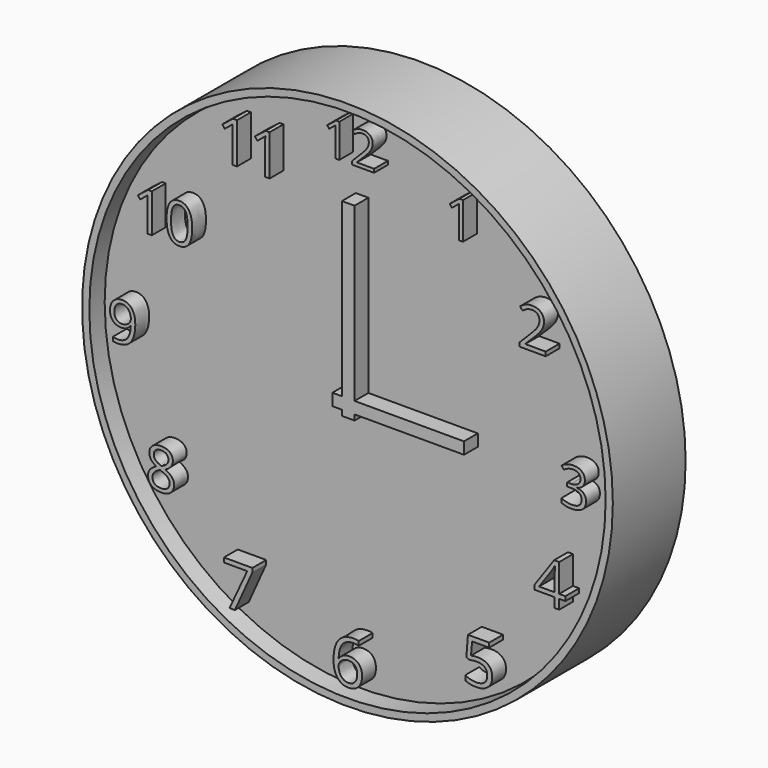
from build123d import *

# Parameters (mm, degrees)
F0_R            = 74.0699095202
F0_R_2          = 72.0569454693
F1_DEPTH        = 25.4
F2_R            = 71.6288838852
F3_DEPTH        = 20.574
F4_TEXT_SIZE    = 13.134137003
F4_TEXT_SIZE_2  = 14.3281546318
F4_TEXT_SIZE_3  = 15.5221670866
F4_TEXT_SIZE_4  = 14.7261585678
F4_TEXT_SIZE_5  = 16.3181736651
F4_TEXT_SIZE_6  = 16.7161795414
F4_TEXT_SIZE_7  = 16.7161847154
F4_TEXT_SIZE_8  = 15.5221722606
F4_TEXT_SIZE_9  = 15.1241631506
F4_TEXT_SIZE_10 = 15.1241612103
F4_TEXT_SIZE_11 = 15.9201729629
F4_TEXT_SIZE_12 = 17.1141854177
F5_DEPTH        = 25.4
F6_W            = 3.5199410049
F6_H            = 1.5269855503
F6_W_2          = 2.6841056533
F6_H_2          = 3.2999463147
F6_W_3          = 30.535359052
F6_H_3          = 47.972215456
F7_DEPTH        = 25.4


# Not quite as in the source:
# - Text() gives the source's letters only with a copy of the font that has no kerning and outlines rounded to 1/6400 em; it was checked with that copy


with BuildPart() as f1:
    # F0 (on Front) → F1 (new body)
    with BuildSketch(Plane.XZ):
        Circle(F0_R)
        Circle(F0_R_2, mode=Mode.SUBTRACT)
    extrude(amount=F1_DEPTH)


with BuildPart() as f3:
    # F2 (on Front) → F3 (new body)
    with BuildSketch(Plane.XZ):
        Circle(F2_R)
    extrude(amount=F3_DEPTH)

    # F4 (on Front) → F5 (join)
    with BuildSketch(Plane.XZ):
        with Locations((-6.8775145337, 59.4618432224)):
            Text('12', F4_TEXT_SIZE, font='Open Sans', text_align=(TextAlign.LEFT, TextAlign.BOTTOM))
        with Locations((27.2234939039, 50.5783893168)):
            Text('1', F4_TEXT_SIZE_2, font='Open Sans', text_align=(TextAlign.LEFT, TextAlign.BOTTOM))
        with Locations((47.2829155624, 29.9458447844)):
            Text('2', F4_TEXT_SIZE_3, font='Open Sans', text_align=(TextAlign.LEFT, TextAlign.BOTTOM))
        with Locations((59.0320006013, -5.0148512237)):
            Text('3', F4_TEXT_SIZE_4, font='Open Sans', text_align=(TextAlign.LEFT, TextAlign.BOTTOM))
        with Locations((51.8073847343, -31.0920923948)):
            Text('4', F4_TEXT_SIZE_5, font='Open Sans', text_align=(TextAlign.LEFT, TextAlign.BOTTOM))
        with Locations((31.8085066974, -57.4558973312)):
            Text('5', F4_TEXT_SIZE_6, font='Open Sans', text_align=(TextAlign.LEFT, TextAlign.BOTTOM))
        with Locations((-35.2472625673, -60.6080964208)):
            Text('7', F4_TEXT_SIZE_7, font='Open Sans', text_align=(TextAlign.LEFT, TextAlign.BOTTOM))
        with Locations((-56.4529299736, -38.2561739534)):
            Text('8', F4_TEXT_SIZE_8, font='Open Sans', text_align=(TextAlign.LEFT, TextAlign.BOTTOM))
        with Locations((-67.0557618141, -5.5879778229)):
            Text('9', F4_TEXT_SIZE_9, font='Open Sans', text_align=(TextAlign.LEFT, TextAlign.BOTTOM))
        with Locations((-59.8916858435, 23.9280257374)):
            Text('10', F4_TEXT_SIZE_10, font='Open Sans', text_align=(TextAlign.LEFT, TextAlign.BOTTOM))
        with Locations((-36.3935157657, 48.5724471509)):
            Text('11', F4_TEXT_SIZE_11, font='Open Sans', text_align=(TextAlign.LEFT, TextAlign.BOTTOM))
        with Locations((-4.8715728335, -69.2049860954)):
            Text('6', F4_TEXT_SIZE_12, font='Open Sans', text_align=(TextAlign.LEFT, TextAlign.BOTTOM))
    extrude(amount=F5_DEPTH)

    # F6 (on Front) → F7 (join)
    with BuildSketch(Plane.XZ):
        with Locations((0.2199950977, -2.4264553795)):
            Rectangle(F6_W, F6_H)
        with Locations((-2.8820282314, -0.012989447)):
            Rectangle(F6_W_2, F6_H_2)
        with Locations((0.2199950977, -0.012989447)):
            Rectangle(F6_W, F6_H_2)
        with Locations((17.2476451262, -0.012989447)):
            Rectangle(F6_W_3, F6_H_2)
        with Locations((0.2199950977, 25.6230914383)):
            Rectangle(F6_W, F6_H_3)
    extrude(amount=F7_DEPTH)


solid = Compound([f1.part, f3.part])
